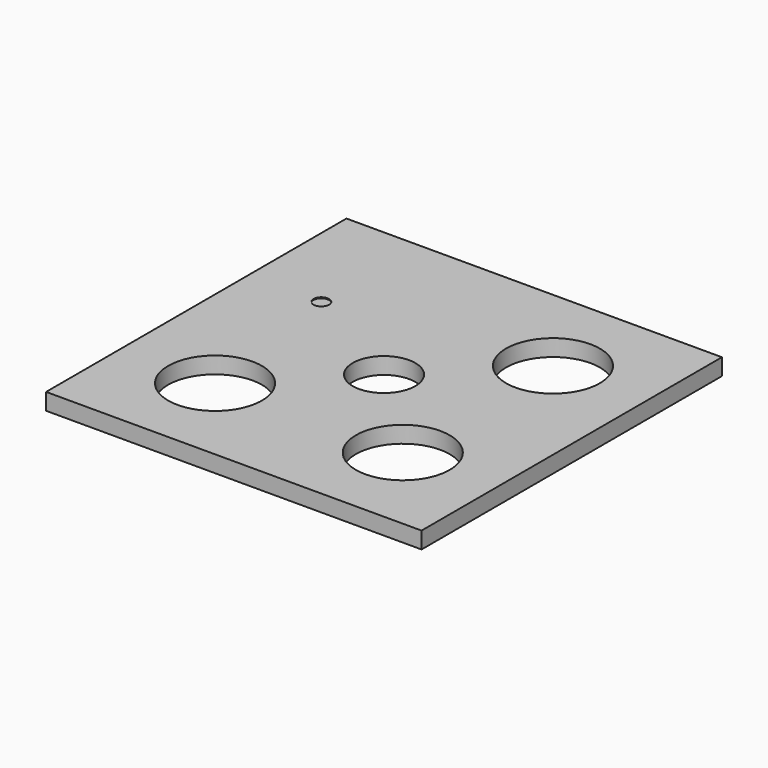
from build123d import *

# Parameters (mm, degrees)
F0_R     = 1.5875
F1_DEPTH = 3.3782
F2_D     = 19.05
F3_D     = 12.7
F4_DEPTH = 3.175


# Not quite as in the source:
# - a feature names something its author has since deleted; it is built from what else it names


with BuildPart() as f1:
    # F0 (on Top) → F1 (new body)
    with BuildSketch(Plane.XY):
        Polygon((38.1, 38.1), (-38.1, 38.1), (-38.1, -38.1), (0, -38.1), (38.1, -38.1), (38.1, 0), align=None)
        with Locations((-23.3484897763, 13.2784806192)):
            Circle(F0_R, mode=Mode.SUBTRACT)
    extrude(amount=F1_DEPTH)

    # F2 (through all)
    with Locations(Plane(origin=(0, 0, 0), x_dir=(1, 0, 0), z_dir=(0, 0, -1))):
        with Locations((19.05, -19.05), (19.05, 19.05), (-19.05, 19.05)):
            Hole(F2_D / 2)

    # F3 (through all)
    with Locations(Plane(origin=(0, 0, 0), x_dir=(1, 0, 0), z_dir=(0, 0, -1))):
        with Locations((0, 0)):
            Hole(F3_D / 2)

    # F0 (on Top) → F4 (join, symmetric)
    with BuildSketch(Plane.XY):
        with Locations((-23.3484897763, 13.2784806192)):
            Circle(F0_R)
    extrude(amount=F4_DEPTH, both=True)


solid = f1.part
